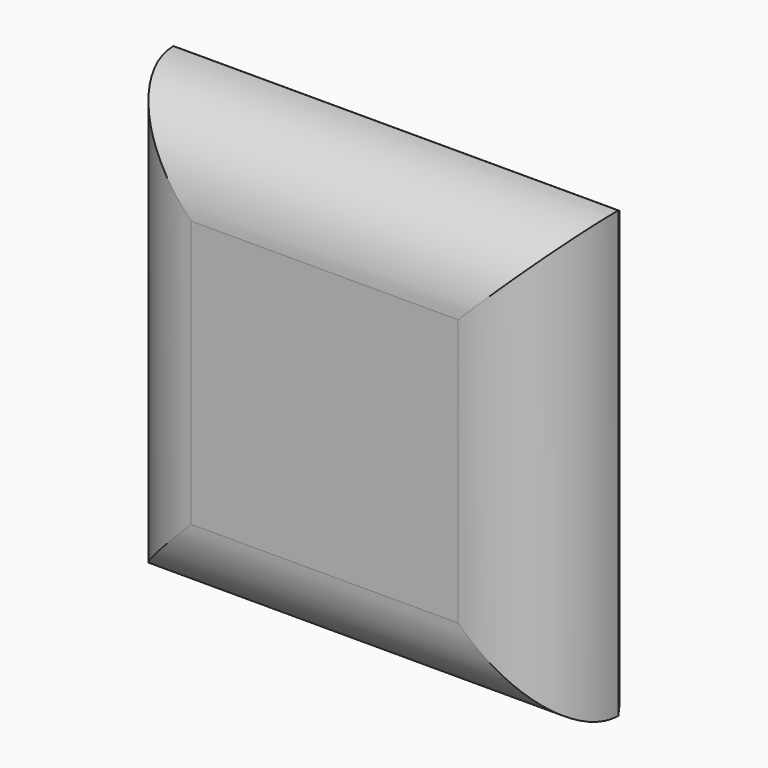
from build123d import *

# Parameters (mm, degrees)
F0_W        = 25.4
F0_H        = 25.4
F1_DEPTH    = 7.62
F2_R        = 5.08
F3_T1_DEPTH = 47.3970452561
F3_T3_DEPTH = 47.3970452561


# Not quite as in the source:
# - a fillet or chamfer that OpenCascade refuses, or shapes differently, is made with other operations: its cross-section is extruded or revolved along the edge and cut away or added


with BuildPart() as f1:
    # F0 (on Front) → F1 (new body)
    with BuildSketch(Plane.XZ):
        Rectangle(F0_W, F0_H)
    extrude(amount=F1_DEPTH)

    # F2
    f2_edges = [f1.edges().sort_by_distance(p)[0] for p in [
        (0, -7.62, 12.7),
        (-12.7, -7.62, 0),
        (12.7, -7.62, 0),
        (0, -7.62, -12.7),
    ]]
    fillet(f2_edges, radius=F2_R)

    # F3: fillet of radius 5.08 on 4 edges, made by hand

    # F3_s2 → F3_t1 (cut)
    with BuildSketch(Plane.YZ.offset(-23.6985226281)):
        with BuildLine():
            ThreePointArc((-2.54, -12.7), (-0.6805909488, -10.8405909488), (0, -8.3005909488))
            Line((0, -8.3005909488), (0, -12.7))
            Line((0, -12.7), (-2.54, -12.7))
        make_face()
        with BuildLine():
            ThreePointArc((0, 8.3005909488), (-0.6805909488, 10.8405909488), (-2.54, 12.7))
            Line((-2.54, 12.7), (0, 12.7))
            Line((0, 12.7), (0, 8.3005909488))
        make_face()
    extrude(amount=F3_T1_DEPTH, mode=Mode.SUBTRACT)

    # F3_s4 → F3_t3 (cut)
    with BuildSketch(Plane.XY.offset(-23.6985226281)):
        with BuildLine():
            ThreePointArc((-8.3005909488, 0), (-10.8405909488, -0.6805909488), (-12.7, -2.54))
            Line((-12.7, -2.54), (-12.7, 0))
            Line((-12.7, 0), (-8.3005909488, 0))
        make_face()
        with BuildLine():
            ThreePointArc((12.7, -2.54), (10.8405909488, -0.6805909488), (8.3005909488, 0))
            Line((8.3005909488, 0), (12.7, 0))
            Line((12.7, 0), (12.7, -2.54))
        make_face()
    extrude(amount=F3_T3_DEPTH, mode=Mode.SUBTRACT)


solid = f1.part
